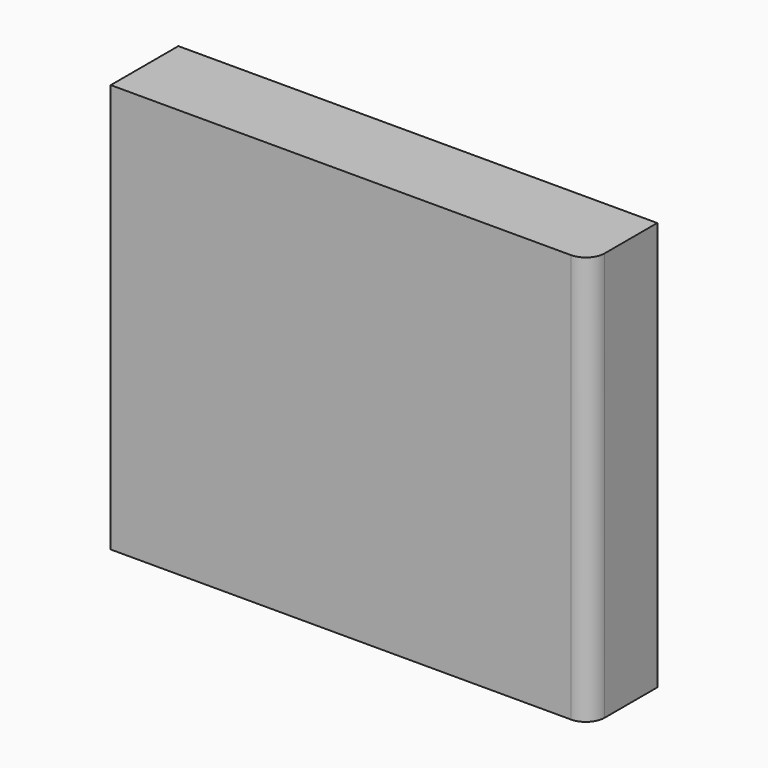
from build123d import *

# Parameters (mm, degrees)
F0_W     = 255.0496831536
F0_H     = 217.740483582
F1_DEPTH = 45
F2_R     = 10


# Not quite as in the source:
# - the program builds the solid bodies; features that only make, move or delete a surface that nothing else refers to are left out


with BuildPart() as f1:
    # F0 (on Front) → F1 (new body)
    with BuildSketch(Plane.XZ):
        with Locations((-30.0156064332, 34.8116643727)):
            Rectangle(F0_W, F0_H)
    extrude(amount=F1_DEPTH)

    # F2
    f2_edges = [f1.edges().sort_by_distance(p)[0] for p in [
        (97.509235, -45, 34.811664),
    ]]
    fillet(f2_edges, radius=F2_R)


solid = f1.part
